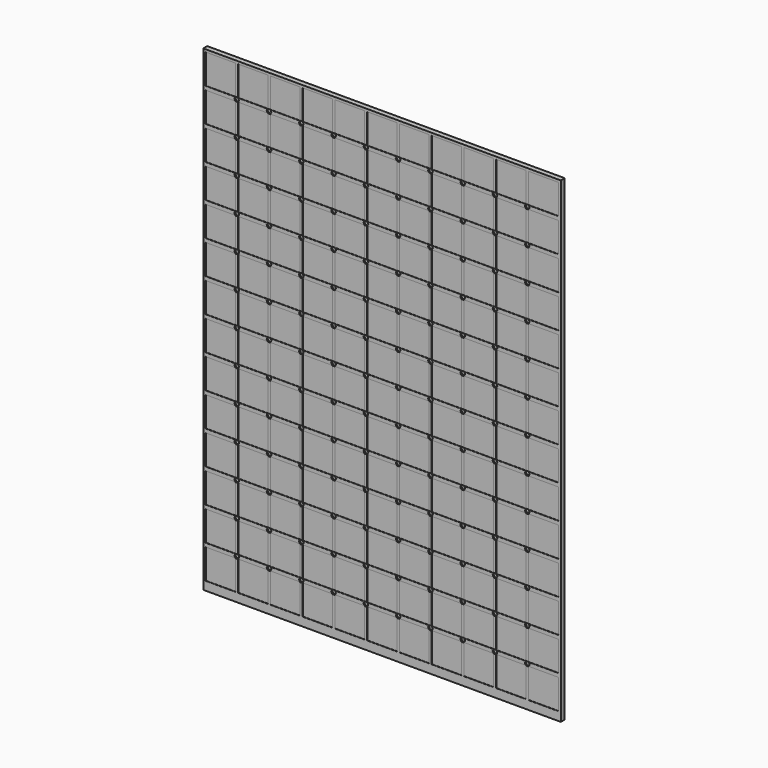
from build123d import *

# Parameters (mm, degrees)
F0_W     = 1828.8
F0_H     = 2438.4
F1_DEPTH = 25.4
F2_W     = 152.4
F2_H     = 152.4
F3_DEPTH = 1.5875
F5_DEPTH = 6.35


# Not quite as in the source:
# - a length typed as a fraction of an inch, garbled in the dataset ("3 / 203.2 mm" for 3/8 in), is restored


with BuildPart() as f1:
    # F0 (on Front) → F1 (new body)
    with BuildSketch(Plane.XZ):
        with Locations((816.0034323931, 1150.0703020215)):
            Rectangle(F0_W, F0_H)
    extrude(amount=F1_DEPTH)

    # F2 (on face) → F3 (cut)
    with BuildSketch(Plane.XZ.offset(25.4)):
        with Locations((-9.4965676069, 2280.3703020215)):
            Rectangle(F2_W, F2_H)
        with Locations((-9.4965676069, 2108.9203020215)):
            Rectangle(F2_W, F2_H)
        with Locations((-9.4965676069, 1937.4703020215)):
            Rectangle(F2_W, F2_H)
        with Locations((-9.4965676069, 1766.0203020215)):
            Rectangle(F2_W, F2_H)
        with Locations((-9.4965676069, 1594.5703020215)):
            Rectangle(F2_W, F2_H)
        with Locations((-9.4965676069, 1423.1203020215)):
            Rectangle(F2_W, F2_H)
        with Locations((-9.4965676069, 1251.6703020215)):
            Rectangle(F2_W, F2_H)
        with Locations((-9.4965676069, 1080.2203020215)):
            Rectangle(F2_W, F2_H)
        with Locations((155.6034323931, 2280.3703020215)):
            Rectangle(F2_W, F2_H)
        with Locations((155.6034323931, 2108.9203020215)):
            Rectangle(F2_W, F2_H)
        with Locations((155.6034323931, 1937.4703020215)):
            Rectangle(F2_W, F2_H)
        with Locations((155.6034323931, 1766.0203020215)):
            Rectangle(F2_W, F2_H)
        with Locations((155.6034323931, 1594.5703020215)):
            Rectangle(F2_W, F2_H)
        with Locations((155.6034323931, 1423.1203020215)):
            Rectangle(F2_W, F2_H)
        with Locations((155.6034323931, 1251.6703020215)):
            Rectangle(F2_W, F2_H)
        with Locations((155.6034323931, 1080.2203020215)):
            Rectangle(F2_W, F2_H)
        with Locations((320.7034323931, 2280.3703020215)):
            Rectangle(F2_W, F2_H)
        with Locations((320.7034323931, 2108.9203020215)):
            Rectangle(F2_W, F2_H)
        with Locations((320.7034323931, 1937.4703020215)):
            Rectangle(F2_W, F2_H)
        with Locations((320.7034323931, 1766.0203020215)):
            Rectangle(F2_W, F2_H)
        with Locations((320.7034323931, 1594.5703020215)):
            Rectangle(F2_W, F2_H)
        with Locations((320.7034323931, 1423.1203020215)):
            Rectangle(F2_W, F2_H)
        with Locations((320.7034323931, 1251.6703020215)):
            Rectangle(F2_W, F2_H)
        with Locations((320.7034323931, 1080.2203020215)):
            Rectangle(F2_W, F2_H)
        with Locations((485.8034323931, 2280.3703020215)):
            Rectangle(F2_W, F2_H)
        with Locations((485.8034323931, 2108.9203020215)):
            Rectangle(F2_W, F2_H)
        with Locations((485.8034323931, 1937.4703020215)):
            Rectangle(F2_W, F2_H)
        with Locations((485.8034323931, 1766.0203020215)):
            Rectangle(F2_W, F2_H)
        with Locations((485.8034323931, 1594.5703020215)):
            Rectangle(F2_W, F2_H)
        with Locations((485.8034323931, 1423.1203020215)):
            Rectangle(F2_W, F2_H)
        with Locations((485.8034323931, 1251.6703020215)):
            Rectangle(F2_W, F2_H)
        with Locations((485.8034323931, 1080.2203020215)):
            Rectangle(F2_W, F2_H)
        with Locations((650.9034323931, 2280.3703020215)):
            Rectangle(F2_W, F2_H)
        with Locations((650.9034323931, 2108.9203020215)):
            Rectangle(F2_W, F2_H)
        with Locations((650.9034323931, 1937.4703020215)):
            Rectangle(F2_W, F2_H)
        with Locations((650.9034323931, 1766.0203020215)):
            Rectangle(F2_W, F2_H)
        with Locations((650.9034323931, 1594.5703020215)):
            Rectangle(F2_W, F2_H)
        with Locations((650.9034323931, 1423.1203020215)):
            Rectangle(F2_W, F2_H)
        with Locations((650.9034323931, 1251.6703020215)):
            Rectangle(F2_W, F2_H)
        with Locations((650.9034323931, 1080.2203020215)):
            Rectangle(F2_W, F2_H)
        with Locations((816.0034323931, 2280.3703020215)):
            Rectangle(F2_W, F2_H)
        with Locations((816.0034323931, 2108.9203020215)):
            Rectangle(F2_W, F2_H)
        with Locations((816.0034323931, 1937.4703020215)):
            Rectangle(F2_W, F2_H)
        with Locations((816.0034323931, 1766.0203020215)):
            Rectangle(F2_W, F2_H)
        with Locations((816.0034323931, 1594.5703020215)):
            Rectangle(F2_W, F2_H)
        with Locations((816.0034323931, 1423.1203020215)):
            Rectangle(F2_W, F2_H)
        with Locations((816.0034323931, 1251.6703020215)):
            Rectangle(F2_W, F2_H)
        with Locations((816.0034323931, 1080.2203020215)):
            Rectangle(F2_W, F2_H)
        with Locations((981.1034323931, 2280.3703020215)):
            Rectangle(F2_W, F2_H)
        with Locations((981.1034323931, 2108.9203020215)):
            Rectangle(F2_W, F2_H)
        with Locations((981.1034323931, 1937.4703020215)):
            Rectangle(F2_W, F2_H)
        with Locations((981.1034323931, 1766.0203020215)):
            Rectangle(F2_W, F2_H)
        with Locations((981.1034323931, 1594.5703020215)):
            Rectangle(F2_W, F2_H)
        with Locations((981.1034323931, 1423.1203020215)):
            Rectangle(F2_W, F2_H)
        with Locations((981.1034323931, 1251.6703020215)):
            Rectangle(F2_W, F2_H)
        with Locations((981.1034323931, 1080.2203020215)):
            Rectangle(F2_W, F2_H)
        with Locations((-9.4965676069, 908.7703020215)):
            Rectangle(F2_W, F2_H)
        with Locations((155.6034323931, 908.7703020215)):
            Rectangle(F2_W, F2_H)
        with Locations((320.7034323931, 908.7703020215)):
            Rectangle(F2_W, F2_H)
        with Locations((485.8034323931, 908.7703020215)):
            Rectangle(F2_W, F2_H)
        with Locations((650.9034323931, 908.7703020215)):
            Rectangle(F2_W, F2_H)
        with Locations((816.0034323931, 908.7703020215)):
            Rectangle(F2_W, F2_H)
        with Locations((981.1034323931, 908.7703020215)):
            Rectangle(F2_W, F2_H)
        with Locations((1146.2034323931, 2280.3703020215)):
            Rectangle(F2_W, F2_H)
        with Locations((1146.2034323931, 2108.9203020215)):
            Rectangle(F2_W, F2_H)
        with Locations((1146.2034323931, 1937.4703020215)):
            Rectangle(F2_W, F2_H)
        with Locations((1146.2034323931, 1766.0203020215)):
            Rectangle(F2_W, F2_H)
        with Locations((1146.2034323931, 1594.5703020215)):
            Rectangle(F2_W, F2_H)
        with Locations((1146.2034323931, 1423.1203020215)):
            Rectangle(F2_W, F2_H)
        with Locations((1146.2034323931, 1251.6703020215)):
            Rectangle(F2_W, F2_H)
        with Locations((1146.2034323931, 1080.2203020215)):
            Rectangle(F2_W, F2_H)
        with Locations((1146.2034323931, 908.7703020215)):
            Rectangle(F2_W, F2_H)
        with Locations((1311.3034323931, 2280.3703020215)):
            Rectangle(F2_W, F2_H)
        with Locations((1311.3034323931, 2108.9203020215)):
            Rectangle(F2_W, F2_H)
        with Locations((1311.3034323931, 1937.4703020215)):
            Rectangle(F2_W, F2_H)
        with Locations((1311.3034323931, 1766.0203020215)):
            Rectangle(F2_W, F2_H)
        with Locations((1311.3034323931, 1594.5703020215)):
            Rectangle(F2_W, F2_H)
        with Locations((1311.3034323931, 1423.1203020215)):
            Rectangle(F2_W, F2_H)
        with Locations((1311.3034323931, 1251.6703020215)):
            Rectangle(F2_W, F2_H)
        with Locations((1311.3034323931, 1080.2203020215)):
            Rectangle(F2_W, F2_H)
        with Locations((1311.3034323931, 908.7703020215)):
            Rectangle(F2_W, F2_H)
        with Locations((1476.4034323931, 2280.3703020215)):
            Rectangle(F2_W, F2_H)
        with Locations((1476.4034323931, 2108.9203020215)):
            Rectangle(F2_W, F2_H)
        with Locations((1476.4034323931, 1937.4703020215)):
            Rectangle(F2_W, F2_H)
        with Locations((1476.4034323931, 1766.0203020215)):
            Rectangle(F2_W, F2_H)
        with Locations((1476.4034323931, 1594.5703020215)):
            Rectangle(F2_W, F2_H)
        with Locations((1476.4034323931, 1423.1203020215)):
            Rectangle(F2_W, F2_H)
        with Locations((1476.4034323931, 1251.6703020215)):
            Rectangle(F2_W, F2_H)
        with Locations((1476.4034323931, 1080.2203020215)):
            Rectangle(F2_W, F2_H)
        with Locations((1476.4034323931, 908.7703020215)):
            Rectangle(F2_W, F2_H)
        with Locations((1641.5034323931, 2280.3703020215)):
            Rectangle(F2_W, F2_H)
        with Locations((1641.5034323931, 2108.9203020215)):
            Rectangle(F2_W, F2_H)
        with Locations((1641.5034323931, 1937.4703020215)):
            Rectangle(F2_W, F2_H)
        with Locations((1641.5034323931, 1766.0203020215)):
            Rectangle(F2_W, F2_H)
        with Locations((1641.5034323931, 1594.5703020215)):
            Rectangle(F2_W, F2_H)
        with Locations((1641.5034323931, 1423.1203020215)):
            Rectangle(F2_W, F2_H)
        with Locations((1641.5034323931, 1251.6703020215)):
            Rectangle(F2_W, F2_H)
        with Locations((1641.5034323931, 1080.2203020215)):
            Rectangle(F2_W, F2_H)
        with Locations((1641.5034323931, 908.7703020215)):
            Rectangle(F2_W, F2_H)
        with Locations((-9.4965676069, 737.3203020215)):
            Rectangle(F2_W, F2_H)
        with Locations((-9.4965676069, 565.8703020215)):
            Rectangle(F2_W, F2_H)
        with Locations((-9.4965676069, 394.4203020215)):
            Rectangle(F2_W, F2_H)
        with Locations((-9.4965676069, 222.9703020215)):
            Rectangle(F2_W, F2_H)
        with Locations((-9.4965676069, 51.5203020215)):
            Rectangle(F2_W, F2_H)
        with Locations((155.6034323931, 737.3203020215)):
            Rectangle(F2_W, F2_H)
        with Locations((155.6034323931, 565.8703020215)):
            Rectangle(F2_W, F2_H)
        with Locations((155.6034323931, 394.4203020215)):
            Rectangle(F2_W, F2_H)
        with Locations((155.6034323931, 222.9703020215)):
            Rectangle(F2_W, F2_H)
        with Locations((155.6034323931, 51.5203020215)):
            Rectangle(F2_W, F2_H)
        with Locations((320.7034323931, 737.3203020215)):
            Rectangle(F2_W, F2_H)
        with Locations((320.7034323931, 565.8703020215)):
            Rectangle(F2_W, F2_H)
        with Locations((320.7034323931, 394.4203020215)):
            Rectangle(F2_W, F2_H)
        with Locations((320.7034323931, 222.9703020215)):
            Rectangle(F2_W, F2_H)
        with Locations((320.7034323931, 51.5203020215)):
            Rectangle(F2_W, F2_H)
        with Locations((485.8034323931, 737.3203020215)):
            Rectangle(F2_W, F2_H)
        with Locations((485.8034323931, 565.8703020215)):
            Rectangle(F2_W, F2_H)
        with Locations((485.8034323931, 394.4203020215)):
            Rectangle(F2_W, F2_H)
        with Locations((485.8034323931, 222.9703020215)):
            Rectangle(F2_W, F2_H)
        with Locations((485.8034323931, 51.5203020215)):
            Rectangle(F2_W, F2_H)
        with Locations((650.9034323931, 737.3203020215)):
            Rectangle(F2_W, F2_H)
        with Locations((650.9034323931, 565.8703020215)):
            Rectangle(F2_W, F2_H)
        with Locations((650.9034323931, 394.4203020215)):
            Rectangle(F2_W, F2_H)
        with Locations((650.9034323931, 222.9703020215)):
            Rectangle(F2_W, F2_H)
        with Locations((650.9034323931, 51.5203020215)):
            Rectangle(F2_W, F2_H)
        with Locations((816.0034323931, 737.3203020215)):
            Rectangle(F2_W, F2_H)
        with Locations((816.0034323931, 565.8703020215)):
            Rectangle(F2_W, F2_H)
        with Locations((816.0034323931, 394.4203020215)):
            Rectangle(F2_W, F2_H)
        with Locations((816.0034323931, 222.9703020215)):
            Rectangle(F2_W, F2_H)
        with Locations((816.0034323931, 51.5203020215)):
            Rectangle(F2_W, F2_H)
        with Locations((981.1034323931, 737.3203020215)):
            Rectangle(F2_W, F2_H)
        with Locations((981.1034323931, 565.8703020215)):
            Rectangle(F2_W, F2_H)
        with Locations((981.1034323931, 394.4203020215)):
            Rectangle(F2_W, F2_H)
        with Locations((981.1034323931, 222.9703020215)):
            Rectangle(F2_W, F2_H)
        with Locations((981.1034323931, 51.5203020215)):
            Rectangle(F2_W, F2_H)
        with Locations((1146.2034323931, 737.3203020215)):
            Rectangle(F2_W, F2_H)
        with Locations((1146.2034323931, 565.8703020215)):
            Rectangle(F2_W, F2_H)
        with Locations((1146.2034323931, 394.4203020215)):
            Rectangle(F2_W, F2_H)
        with Locations((1146.2034323931, 222.9703020215)):
            Rectangle(F2_W, F2_H)
        with Locations((1146.2034323931, 51.5203020215)):
            Rectangle(F2_W, F2_H)
        with Locations((1311.3034323931, 737.3203020215)):
            Rectangle(F2_W, F2_H)
        with Locations((1311.3034323931, 565.8703020215)):
            Rectangle(F2_W, F2_H)
        with Locations((1311.3034323931, 394.4203020215)):
            Rectangle(F2_W, F2_H)
        with Locations((1311.3034323931, 222.9703020215)):
            Rectangle(F2_W, F2_H)
        with Locations((1311.3034323931, 51.5203020215)):
            Rectangle(F2_W, F2_H)
        with Locations((1476.4034323931, 737.3203020215)):
            Rectangle(F2_W, F2_H)
        with Locations((1476.4034323931, 565.8703020215)):
            Rectangle(F2_W, F2_H)
        with Locations((1476.4034323931, 394.4203020215)):
            Rectangle(F2_W, F2_H)
        with Locations((1476.4034323931, 222.9703020215)):
            Rectangle(F2_W, F2_H)
        with Locations((1476.4034323931, 51.5203020215)):
            Rectangle(F2_W, F2_H)
        with Locations((1641.5034323931, 737.3203020215)):
            Rectangle(F2_W, F2_H)
        with Locations((1641.5034323931, 565.8703020215)):
            Rectangle(F2_W, F2_H)
        with Locations((1641.5034323931, 394.4203020215)):
            Rectangle(F2_W, F2_H)
        with Locations((1641.5034323931, 222.9703020215)):
            Rectangle(F2_W, F2_H)
        with Locations((1641.5034323931, 51.5203020215)):
            Rectangle(F2_W, F2_H)
    extrude(amount=-F3_DEPTH, mode=Mode.SUBTRACT)

    # F4 (on face) → F5 (cut)
    with BuildSketch(Plane.XZ.offset(25.4)):
        Polygon((66.8225524701, 2183.8503020215), (79.2843123161, 2183.8503020215), (85.5151922391, 2194.642502624), (79.2843123161, 2205.4347032265), (66.8225524701, 2205.4347032265), (60.5916725471, 2194.642502624), align=None)
        Polygon((79.2843123161, 2033.9847032265), (66.8225524701, 2033.9847032265), (60.5916725471, 2023.192502624), (66.8225524701, 2012.4003020215), (79.2843123161, 2012.4003020215), (85.5151922391, 2023.192502624), align=None)
        Polygon((79.2843123161, 1862.5347032265), (66.8225524701, 1862.5347032265), (60.5916725471, 1851.742502624), (66.8225524701, 1840.9503020215), (79.2843123161, 1840.9503020215), (85.5151922391, 1851.742502624), align=None)
        Polygon((79.2843123161, 1691.0847032265), (66.8225524701, 1691.0847032265), (60.5916725471, 1680.292502624), (66.8225524701, 1669.5003020215), (79.2843123161, 1669.5003020215), (85.5151922391, 1680.292502624), align=None)
        Polygon((79.2843123161, 1519.6347032265), (66.8225524701, 1519.6347032265), (60.5916725471, 1508.842502624), (66.8225524701, 1498.0503020215), (79.2843123161, 1498.0503020215), (85.5151922391, 1508.842502624), align=None)
        Polygon((79.2843123161, 1348.1847032265), (66.8225524701, 1348.1847032265), (60.5916725471, 1337.392502624), (66.8225524701, 1326.6003020215), (79.2843123161, 1326.6003020215), (85.5151922391, 1337.392502624), align=None)
        Polygon((79.2843123161, 1176.7347032265), (66.8225524701, 1176.7347032265), (60.5916725471, 1165.942502624), (66.8225524701, 1155.1503020215), (79.2843123161, 1155.1503020215), (85.5151922391, 1165.942502624), align=None)
        Polygon((79.2843123161, 1005.2847032265), (66.8225524701, 1005.2847032265), (60.5916725471, 994.492502624), (66.8225524701, 983.7003020215), (79.2843123161, 983.7003020215), (85.5151922391, 994.492502624), align=None)
        Polygon((244.3843123161, 2205.4347032265), (231.9225524701, 2205.4347032265), (225.6916725471, 2194.642502624), (231.9225524701, 2183.8503020215), (244.3843123161, 2183.8503020215), (250.6151922391, 2194.642502624), align=None)
        Polygon((244.3843123161, 2033.9847032265), (231.9225524701, 2033.9847032265), (225.6916725471, 2023.192502624), (231.9225524701, 2012.4003020215), (244.3843123161, 2012.4003020215), (250.6151922391, 2023.192502624), align=None)
        Polygon((244.3843123161, 1862.5347032265), (231.9225524701, 1862.5347032265), (225.6916725471, 1851.742502624), (231.9225524701, 1840.9503020215), (244.3843123161, 1840.9503020215), (250.6151922391, 1851.742502624), align=None)
        Polygon((244.3843123161, 1691.0847032265), (231.9225524701, 1691.0847032265), (225.6916725471, 1680.292502624), (231.9225524701, 1669.5003020215), (244.3843123161, 1669.5003020215), (250.6151922391, 1680.292502624), align=None)
        Polygon((244.3843123161, 1519.6347032265), (231.9225524701, 1519.6347032265), (225.6916725471, 1508.842502624), (231.9225524701, 1498.0503020215), (244.3843123161, 1498.0503020215), (250.6151922391, 1508.842502624), align=None)
        Polygon((244.3843123161, 1348.1847032265), (231.9225524701, 1348.1847032265), (225.6916725471, 1337.392502624), (231.9225524701, 1326.6003020215), (244.3843123161, 1326.6003020215), (250.6151922391, 1337.392502624), align=None)
        Polygon((244.3843123161, 1176.7347032265), (231.9225524701, 1176.7347032265), (225.6916725471, 1165.942502624), (231.9225524701, 1155.1503020215), (244.3843123161, 1155.1503020215), (250.6151922391, 1165.942502624), align=None)
        Polygon((244.3843123161, 1005.2847032265), (231.9225524701, 1005.2847032265), (225.6916725471, 994.492502624), (231.9225524701, 983.7003020215), (244.3843123161, 983.7003020215), (250.6151922391, 994.492502624), align=None)
        Polygon((409.4843123161, 2205.4347032265), (397.0225524701, 2205.4347032265), (390.7916725471, 2194.642502624), (397.0225524701, 2183.8503020215), (409.4843123161, 2183.8503020215), (415.7151922391, 2194.642502624), align=None)
        Polygon((409.4843123161, 2033.9847032265), (397.0225524701, 2033.9847032265), (390.7916725471, 2023.192502624), (397.0225524701, 2012.4003020215), (409.4843123161, 2012.4003020215), (415.7151922391, 2023.192502624), align=None)
        Polygon((409.4843123161, 1862.5347032265), (397.0225524701, 1862.5347032265), (390.7916725471, 1851.742502624), (397.0225524701, 1840.9503020215), (409.4843123161, 1840.9503020215), (415.7151922391, 1851.742502624), align=None)
        Polygon((409.4843123161, 1691.0847032265), (397.0225524701, 1691.0847032265), (390.7916725471, 1680.292502624), (397.0225524701, 1669.5003020215), (409.4843123161, 1669.5003020215), (415.7151922391, 1680.292502624), align=None)
        Polygon((409.4843123161, 1519.6347032265), (397.0225524701, 1519.6347032265), (390.7916725471, 1508.842502624), (397.0225524701, 1498.0503020215), (409.4843123161, 1498.0503020215), (415.7151922391, 1508.842502624), align=None)
        Polygon((409.4843123161, 1348.1847032265), (397.0225524701, 1348.1847032265), (390.7916725471, 1337.392502624), (397.0225524701, 1326.6003020215), (409.4843123161, 1326.6003020215), (415.7151922391, 1337.392502624), align=None)
        Polygon((409.4843123161, 1176.7347032265), (397.0225524701, 1176.7347032265), (390.7916725471, 1165.942502624), (397.0225524701, 1155.1503020215), (409.4843123161, 1155.1503020215), (415.7151922391, 1165.942502624), align=None)
        Polygon((409.4843123161, 1005.2847032265), (397.0225524701, 1005.2847032265), (390.7916725471, 994.492502624), (397.0225524701, 983.7003020215), (409.4843123161, 983.7003020215), (415.7151922391, 994.492502624), align=None)
        Polygon((574.5843123161, 2205.4347032265), (562.1225524701, 2205.4347032265), (555.8916725471, 2194.642502624), (562.1225524701, 2183.8503020215), (574.5843123161, 2183.8503020215), (580.8151922391, 2194.642502624), align=None)
        Polygon((574.5843123161, 2033.9847032265), (562.1225524701, 2033.9847032265), (555.8916725471, 2023.192502624), (562.1225524701, 2012.4003020215), (574.5843123161, 2012.4003020215), (580.8151922391, 2023.192502624), align=None)
        Polygon((574.5843123161, 1862.5347032265), (562.1225524701, 1862.5347032265), (555.8916725471, 1851.742502624), (562.1225524701, 1840.9503020215), (574.5843123161, 1840.9503020215), (580.8151922391, 1851.742502624), align=None)
        Polygon((574.5843123161, 1691.0847032265), (562.1225524701, 1691.0847032265), (555.8916725471, 1680.292502624), (562.1225524701, 1669.5003020215), (574.5843123161, 1669.5003020215), (580.8151922391, 1680.292502624), align=None)
        Polygon((574.5843123161, 1519.6347032265), (562.1225524701, 1519.6347032265), (555.8916725471, 1508.842502624), (562.1225524701, 1498.0503020215), (574.5843123161, 1498.0503020215), (580.8151922391, 1508.842502624), align=None)
        Polygon((574.5843123161, 1348.1847032265), (562.1225524701, 1348.1847032265), (555.8916725471, 1337.392502624), (562.1225524701, 1326.6003020215), (574.5843123161, 1326.6003020215), (580.8151922391, 1337.392502624), align=None)
        Polygon((574.5843123161, 1176.7347032265), (562.1225524701, 1176.7347032265), (555.8916725471, 1165.942502624), (562.1225524701, 1155.1503020215), (574.5843123161, 1155.1503020215), (580.8151922391, 1165.942502624), align=None)
        Polygon((574.5843123161, 1005.2847032265), (562.1225524701, 1005.2847032265), (555.8916725471, 994.492502624), (562.1225524701, 983.7003020215), (574.5843123161, 983.7003020215), (580.8151922391, 994.492502624), align=None)
        Polygon((739.6843123161, 2205.4347032265), (727.2225524701, 2205.4347032265), (720.9916725471, 2194.642502624), (727.2225524701, 2183.8503020215), (739.6843123161, 2183.8503020215), (745.9151922391, 2194.642502624), align=None)
        Polygon((739.6843123161, 2033.9847032265), (727.2225524701, 2033.9847032265), (720.9916725471, 2023.192502624), (727.2225524701, 2012.4003020215), (739.6843123161, 2012.4003020215), (745.9151922391, 2023.192502624), align=None)
        Polygon((739.6843123161, 1862.5347032265), (727.2225524701, 1862.5347032265), (720.9916725471, 1851.742502624), (727.2225524701, 1840.9503020215), (739.6843123161, 1840.9503020215), (745.9151922391, 1851.742502624), align=None)
        Polygon((739.6843123161, 1691.0847032265), (727.2225524701, 1691.0847032265), (720.9916725471, 1680.292502624), (727.2225524701, 1669.5003020215), (739.6843123161, 1669.5003020215), (745.9151922391, 1680.292502624), align=None)
        Polygon((739.6843123161, 1519.6347032265), (727.2225524701, 1519.6347032265), (720.9916725471, 1508.842502624), (727.2225524701, 1498.0503020215), (739.6843123161, 1498.0503020215), (745.9151922391, 1508.842502624), align=None)
        Polygon((739.6843123161, 1348.1847032265), (727.2225524701, 1348.1847032265), (720.9916725471, 1337.392502624), (727.2225524701, 1326.6003020215), (739.6843123161, 1326.6003020215), (745.9151922391, 1337.392502624), align=None)
        Polygon((739.6843123161, 1176.7347032265), (727.2225524701, 1176.7347032265), (720.9916725471, 1165.942502624), (727.2225524701, 1155.1503020215), (739.6843123161, 1155.1503020215), (745.9151922391, 1165.942502624), align=None)
        Polygon((739.6843123161, 1005.2847032265), (727.2225524701, 1005.2847032265), (720.9916725471, 994.492502624), (727.2225524701, 983.7003020215), (739.6843123161, 983.7003020215), (745.9151922391, 994.492502624), align=None)
        Polygon((904.7843123161, 2205.4347032265), (892.3225524701, 2205.4347032265), (886.0916725471, 2194.642502624), (892.3225524701, 2183.8503020215), (904.7843123161, 2183.8503020215), (911.0151922391, 2194.642502624), align=None)
        Polygon((904.7843123161, 2033.9847032265), (892.3225524701, 2033.9847032265), (886.0916725471, 2023.192502624), (892.3225524701, 2012.4003020215), (904.7843123161, 2012.4003020215), (911.0151922391, 2023.192502624), align=None)
        Polygon((904.7843123161, 1862.5347032265), (892.3225524701, 1862.5347032265), (886.0916725471, 1851.742502624), (892.3225524701, 1840.9503020215), (904.7843123161, 1840.9503020215), (911.0151922391, 1851.742502624), align=None)
        Polygon((904.7843123161, 1691.0847032265), (892.3225524701, 1691.0847032265), (886.0916725471, 1680.292502624), (892.3225524701, 1669.5003020215), (904.7843123161, 1669.5003020215), (911.0151922391, 1680.292502624), align=None)
        Polygon((904.7843123161, 1519.6347032265), (892.3225524701, 1519.6347032265), (886.0916725471, 1508.842502624), (892.3225524701, 1498.0503020215), (904.7843123161, 1498.0503020215), (911.0151922391, 1508.842502624), align=None)
        Polygon((904.7843123161, 1348.1847032265), (892.3225524701, 1348.1847032265), (886.0916725471, 1337.392502624), (892.3225524701, 1326.6003020215), (904.7843123161, 1326.6003020215), (911.0151922391, 1337.392502624), align=None)
        Polygon((904.7843123161, 1176.7347032265), (892.3225524701, 1176.7347032265), (886.0916725471, 1165.942502624), (892.3225524701, 1155.1503020215), (904.7843123161, 1155.1503020215), (911.0151922391, 1165.942502624), align=None)
        Polygon((904.7843123161, 1005.2847032265), (892.3225524701, 1005.2847032265), (886.0916725471, 994.492502624), (892.3225524701, 983.7003020215), (904.7843123161, 983.7003020215), (911.0151922391, 994.492502624), align=None)
        Polygon((1069.8843123161, 2205.4347032265), (1057.4225524701, 2205.4347032265), (1051.1916725471, 2194.642502624), (1057.4225524701, 2183.8503020215), (1069.8843123161, 2183.8503020215), (1076.1151922391, 2194.642502624), align=None)
        Polygon((1069.8843123161, 2033.9847032265), (1057.4225524701, 2033.9847032265), (1051.1916725471, 2023.192502624), (1057.4225524701, 2012.4003020215), (1069.8843123161, 2012.4003020215), (1076.1151922391, 2023.192502624), align=None)
        Polygon((1069.8843123161, 1862.5347032265), (1057.4225524701, 1862.5347032265), (1051.1916725471, 1851.742502624), (1057.4225524701, 1840.9503020215), (1069.8843123161, 1840.9503020215), (1076.1151922391, 1851.742502624), align=None)
        Polygon((1069.8843123161, 1691.0847032265), (1057.4225524701, 1691.0847032265), (1051.1916725471, 1680.292502624), (1057.4225524701, 1669.5003020215), (1069.8843123161, 1669.5003020215), (1076.1151922391, 1680.292502624), align=None)
        Polygon((1069.8843123161, 1519.6347032265), (1057.4225524701, 1519.6347032265), (1051.1916725471, 1508.842502624), (1057.4225524701, 1498.0503020215), (1069.8843123161, 1498.0503020215), (1076.1151922391, 1508.842502624), align=None)
        Polygon((1069.8843123161, 1348.1847032265), (1057.4225524701, 1348.1847032265), (1051.1916725471, 1337.392502624), (1057.4225524701, 1326.6003020215), (1069.8843123161, 1326.6003020215), (1076.1151922391, 1337.392502624), align=None)
        Polygon((1069.8843123161, 1176.7347032265), (1057.4225524701, 1176.7347032265), (1051.1916725471, 1165.942502624), (1057.4225524701, 1155.1503020215), (1069.8843123161, 1155.1503020215), (1076.1151922391, 1165.942502624), align=None)
        Polygon((1069.8843123161, 1005.2847032265), (1057.4225524701, 1005.2847032265), (1051.1916725471, 994.492502624), (1057.4225524701, 983.7003020215), (1069.8843123161, 983.7003020215), (1076.1151922391, 994.492502624), align=None)
        Polygon((1234.9843123161, 2205.4347032265), (1222.5225524701, 2205.4347032265), (1216.2916725471, 2194.642502624), (1222.5225524701, 2183.8503020215), (1234.9843123161, 2183.8503020215), (1241.2151922391, 2194.642502624), align=None)
        Polygon((1234.9843123161, 2033.9847032265), (1222.5225524701, 2033.9847032265), (1216.2916725471, 2023.192502624), (1222.5225524701, 2012.4003020215), (1234.9843123161, 2012.4003020215), (1241.2151922391, 2023.192502624), align=None)
        Polygon((1234.9843123161, 1862.5347032265), (1222.5225524701, 1862.5347032265), (1216.2916725471, 1851.742502624), (1222.5225524701, 1840.9503020215), (1234.9843123161, 1840.9503020215), (1241.2151922391, 1851.742502624), align=None)
        Polygon((1234.9843123161, 1691.0847032265), (1222.5225524701, 1691.0847032265), (1216.2916725471, 1680.292502624), (1222.5225524701, 1669.5003020215), (1234.9843123161, 1669.5003020215), (1241.2151922391, 1680.292502624), align=None)
        Polygon((1234.9843123161, 1519.6347032265), (1222.5225524701, 1519.6347032265), (1216.2916725471, 1508.842502624), (1222.5225524701, 1498.0503020215), (1234.9843123161, 1498.0503020215), (1241.2151922391, 1508.842502624), align=None)
        Polygon((1234.9843123161, 1348.1847032265), (1222.5225524701, 1348.1847032265), (1216.2916725471, 1337.392502624), (1222.5225524701, 1326.6003020215), (1234.9843123161, 1326.6003020215), (1241.2151922391, 1337.392502624), align=None)
        Polygon((1234.9843123161, 1176.7347032265), (1222.5225524701, 1176.7347032265), (1216.2916725471, 1165.942502624), (1222.5225524701, 1155.1503020215), (1234.9843123161, 1155.1503020215), (1241.2151922391, 1165.942502624), align=None)
        Polygon((1234.9843123161, 1005.2847032265), (1222.5225524701, 1005.2847032265), (1216.2916725471, 994.492502624), (1222.5225524701, 983.7003020215), (1234.9843123161, 983.7003020215), (1241.2151922391, 994.492502624), align=None)
        Polygon((1400.0843123161, 2205.4347032265), (1387.6225524701, 2205.4347032265), (1381.3916725471, 2194.642502624), (1387.6225524701, 2183.8503020215), (1400.0843123161, 2183.8503020215), (1406.3151922391, 2194.642502624), align=None)
        Polygon((1400.0843123161, 2033.9847032265), (1387.6225524701, 2033.9847032265), (1381.3916725471, 2023.192502624), (1387.6225524701, 2012.4003020215), (1400.0843123161, 2012.4003020215), (1406.3151922391, 2023.192502624), align=None)
        Polygon((1400.0843123161, 1862.5347032265), (1387.6225524701, 1862.5347032265), (1381.3916725471, 1851.742502624), (1387.6225524701, 1840.9503020215), (1400.0843123161, 1840.9503020215), (1406.3151922391, 1851.742502624), align=None)
        Polygon((1400.0843123161, 1691.0847032265), (1387.6225524701, 1691.0847032265), (1381.3916725471, 1680.292502624), (1387.6225524701, 1669.5003020215), (1400.0843123161, 1669.5003020215), (1406.3151922391, 1680.292502624), align=None)
        Polygon((1400.0843123161, 1519.6347032265), (1387.6225524701, 1519.6347032265), (1381.3916725471, 1508.842502624), (1387.6225524701, 1498.0503020215), (1400.0843123161, 1498.0503020215), (1406.3151922391, 1508.842502624), align=None)
        Polygon((1400.0843123161, 1348.1847032265), (1387.6225524701, 1348.1847032265), (1381.3916725471, 1337.392502624), (1387.6225524701, 1326.6003020215), (1400.0843123161, 1326.6003020215), (1406.3151922391, 1337.392502624), align=None)
        Polygon((1400.0843123161, 1176.7347032265), (1387.6225524701, 1176.7347032265), (1381.3916725471, 1165.942502624), (1387.6225524701, 1155.1503020215), (1400.0843123161, 1155.1503020215), (1406.3151922391, 1165.942502624), align=None)
        Polygon((1400.0843123161, 1005.2847032265), (1387.6225524701, 1005.2847032265), (1381.3916725471, 994.492502624), (1387.6225524701, 983.7003020215), (1400.0843123161, 983.7003020215), (1406.3151922391, 994.492502624), align=None)
        Polygon((1565.1843123161, 2205.4347032265), (1552.7225524701, 2205.4347032265), (1546.4916725471, 2194.642502624), (1552.7225524701, 2183.8503020215), (1565.1843123161, 2183.8503020215), (1571.4151922391, 2194.642502624), align=None)
        Polygon((1565.1843123161, 2033.9847032265), (1552.7225524701, 2033.9847032265), (1546.4916725471, 2023.192502624), (1552.7225524701, 2012.4003020215), (1565.1843123161, 2012.4003020215), (1571.4151922391, 2023.192502624), align=None)
        Polygon((1565.1843123161, 1862.5347032265), (1552.7225524701, 1862.5347032265), (1546.4916725471, 1851.742502624), (1552.7225524701, 1840.9503020215), (1565.1843123161, 1840.9503020215), (1571.4151922391, 1851.742502624), align=None)
        Polygon((1565.1843123161, 1691.0847032265), (1552.7225524701, 1691.0847032265), (1546.4916725471, 1680.292502624), (1552.7225524701, 1669.5003020215), (1565.1843123161, 1669.5003020215), (1571.4151922391, 1680.292502624), align=None)
        Polygon((1565.1843123161, 1519.6347032265), (1552.7225524701, 1519.6347032265), (1546.4916725471, 1508.842502624), (1552.7225524701, 1498.0503020215), (1565.1843123161, 1498.0503020215), (1571.4151922391, 1508.842502624), align=None)
        Polygon((1565.1843123161, 1348.1847032265), (1552.7225524701, 1348.1847032265), (1546.4916725471, 1337.392502624), (1552.7225524701, 1326.6003020215), (1565.1843123161, 1326.6003020215), (1571.4151922391, 1337.392502624), align=None)
        Polygon((1565.1843123161, 1176.7347032265), (1552.7225524701, 1176.7347032265), (1546.4916725471, 1165.942502624), (1552.7225524701, 1155.1503020215), (1565.1843123161, 1155.1503020215), (1571.4151922391, 1165.942502624), align=None)
        Polygon((1565.1843123161, 1005.2847032265), (1552.7225524701, 1005.2847032265), (1546.4916725471, 994.492502624), (1552.7225524701, 983.7003020215), (1565.1843123161, 983.7003020215), (1571.4151922391, 994.492502624), align=None)
        Polygon((79.2843123161, 833.8347032265), (66.8225524701, 833.8347032265), (60.5916725471, 823.042502624), (66.8225524701, 812.2503020215), (79.2843123161, 812.2503020215), (85.5151922391, 823.042502624), align=None)
        Polygon((79.2843123161, 662.3847032265), (66.8225524701, 662.3847032265), (60.5916725471, 651.592502624), (66.8225524701, 640.8003020215), (79.2843123161, 640.8003020215), (85.5151922391, 651.592502624), align=None)
        Polygon((79.2843123161, 490.9347032265), (66.8225524701, 490.9347032265), (60.5916725471, 480.142502624), (66.8225524701, 469.3503020215), (79.2843123161, 469.3503020215), (85.5151922391, 480.142502624), align=None)
        Polygon((79.2843123161, 319.4847032265), (66.8225524701, 319.4847032265), (60.5916725471, 308.692502624), (66.8225524701, 297.9003020215), (79.2843123161, 297.9003020215), (85.5151922391, 308.692502624), align=None)
        Polygon((244.3843123161, 833.8347032265), (231.9225524701, 833.8347032265), (225.6916725471, 823.042502624), (231.9225524701, 812.2503020215), (244.3843123161, 812.2503020215), (250.6151922391, 823.042502624), align=None)
        Polygon((244.3843123161, 662.3847032265), (231.9225524701, 662.3847032265), (225.6916725471, 651.592502624), (231.9225524701, 640.8003020215), (244.3843123161, 640.8003020215), (250.6151922391, 651.592502624), align=None)
        Polygon((244.3843123161, 490.9347032265), (231.9225524701, 490.9347032265), (225.6916725471, 480.142502624), (231.9225524701, 469.3503020215), (244.3843123161, 469.3503020215), (250.6151922391, 480.142502624), align=None)
        Polygon((244.3843123161, 319.4847032265), (231.9225524701, 319.4847032265), (225.6916725471, 308.692502624), (231.9225524701, 297.9003020215), (244.3843123161, 297.9003020215), (250.6151922391, 308.692502624), align=None)
        Polygon((409.4843123161, 833.8347032265), (397.0225524701, 833.8347032265), (390.7916725471, 823.042502624), (397.0225524701, 812.2503020215), (409.4843123161, 812.2503020215), (415.7151922391, 823.042502624), align=None)
        Polygon((409.4843123161, 662.3847032265), (397.0225524701, 662.3847032265), (390.7916725471, 651.592502624), (397.0225524701, 640.8003020215), (409.4843123161, 640.8003020215), (415.7151922391, 651.592502624), align=None)
        Polygon((409.4843123161, 490.9347032265), (397.0225524701, 490.9347032265), (390.7916725471, 480.142502624), (397.0225524701, 469.3503020215), (409.4843123161, 469.3503020215), (415.7151922391, 480.142502624), align=None)
        Polygon((409.4843123161, 319.4847032265), (397.0225524701, 319.4847032265), (390.7916725471, 308.692502624), (397.0225524701, 297.9003020215), (409.4843123161, 297.9003020215), (415.7151922391, 308.692502624), align=None)
        Polygon((574.5843123161, 833.8347032265), (562.1225524701, 833.8347032265), (555.8916725471, 823.042502624), (562.1225524701, 812.2503020215), (574.5843123161, 812.2503020215), (580.8151922391, 823.042502624), align=None)
        Polygon((574.5843123161, 662.3847032265), (562.1225524701, 662.3847032265), (555.8916725471, 651.592502624), (562.1225524701, 640.8003020215), (574.5843123161, 640.8003020215), (580.8151922391, 651.592502624), align=None)
        Polygon((574.5843123161, 490.9347032265), (562.1225524701, 490.9347032265), (555.8916725471, 480.142502624), (562.1225524701, 469.3503020215), (574.5843123161, 469.3503020215), (580.8151922391, 480.142502624), align=None)
        Polygon((574.5843123161, 319.4847032265), (562.1225524701, 319.4847032265), (555.8916725471, 308.692502624), (562.1225524701, 297.9003020215), (574.5843123161, 297.9003020215), (580.8151922391, 308.692502624), align=None)
        Polygon((739.6843123161, 833.8347032265), (727.2225524701, 833.8347032265), (720.9916725471, 823.042502624), (727.2225524701, 812.2503020215), (739.6843123161, 812.2503020215), (745.9151922391, 823.042502624), align=None)
        Polygon((739.6843123161, 662.3847032265), (727.2225524701, 662.3847032265), (720.9916725471, 651.592502624), (727.2225524701, 640.8003020215), (739.6843123161, 640.8003020215), (745.9151922391, 651.592502624), align=None)
        Polygon((739.6843123161, 490.9347032265), (727.2225524701, 490.9347032265), (720.9916725471, 480.142502624), (727.2225524701, 469.3503020215), (739.6843123161, 469.3503020215), (745.9151922391, 480.142502624), align=None)
        Polygon((739.6843123161, 319.4847032265), (727.2225524701, 319.4847032265), (720.9916725471, 308.692502624), (727.2225524701, 297.9003020215), (739.6843123161, 297.9003020215), (745.9151922391, 308.692502624), align=None)
        Polygon((904.7843123161, 833.8347032265), (892.3225524701, 833.8347032265), (886.0916725471, 823.042502624), (892.3225524701, 812.2503020215), (904.7843123161, 812.2503020215), (911.0151922391, 823.042502624), align=None)
        Polygon((904.7843123161, 662.3847032265), (892.3225524701, 662.3847032265), (886.0916725471, 651.592502624), (892.3225524701, 640.8003020215), (904.7843123161, 640.8003020215), (911.0151922391, 651.592502624), align=None)
        Polygon((904.7843123161, 490.9347032265), (892.3225524701, 490.9347032265), (886.0916725471, 480.142502624), (892.3225524701, 469.3503020215), (904.7843123161, 469.3503020215), (911.0151922391, 480.142502624), align=None)
        Polygon((904.7843123161, 319.4847032265), (892.3225524701, 319.4847032265), (886.0916725471, 308.692502624), (892.3225524701, 297.9003020215), (904.7843123161, 297.9003020215), (911.0151922391, 308.692502624), align=None)
        Polygon((1069.8843123161, 833.8347032265), (1057.4225524701, 833.8347032265), (1051.1916725471, 823.042502624), (1057.4225524701, 812.2503020215), (1069.8843123161, 812.2503020215), (1076.1151922391, 823.042502624), align=None)
        Polygon((1069.8843123161, 662.3847032265), (1057.4225524701, 662.3847032265), (1051.1916725471, 651.592502624), (1057.4225524701, 640.8003020215), (1069.8843123161, 640.8003020215), (1076.1151922391, 651.592502624), align=None)
        Polygon((1069.8843123161, 490.9347032265), (1057.4225524701, 490.9347032265), (1051.1916725471, 480.142502624), (1057.4225524701, 469.3503020215), (1069.8843123161, 469.3503020215), (1076.1151922391, 480.142502624), align=None)
        Polygon((1069.8843123161, 319.4847032265), (1057.4225524701, 319.4847032265), (1051.1916725471, 308.692502624), (1057.4225524701, 297.9003020215), (1069.8843123161, 297.9003020215), (1076.1151922391, 308.692502624), align=None)
        Polygon((1234.9843123161, 833.8347032265), (1222.5225524701, 833.8347032265), (1216.2916725471, 823.042502624), (1222.5225524701, 812.2503020215), (1234.9843123161, 812.2503020215), (1241.2151922391, 823.042502624), align=None)
        Polygon((1234.9843123161, 662.3847032265), (1222.5225524701, 662.3847032265), (1216.2916725471, 651.592502624), (1222.5225524701, 640.8003020215), (1234.9843123161, 640.8003020215), (1241.2151922391, 651.592502624), align=None)
        Polygon((1234.9843123161, 490.9347032265), (1222.5225524701, 490.9347032265), (1216.2916725471, 480.142502624), (1222.5225524701, 469.3503020215), (1234.9843123161, 469.3503020215), (1241.2151922391, 480.142502624), align=None)
        Polygon((1234.9843123161, 319.4847032265), (1222.5225524701, 319.4847032265), (1216.2916725471, 308.692502624), (1222.5225524701, 297.9003020215), (1234.9843123161, 297.9003020215), (1241.2151922391, 308.692502624), align=None)
        Polygon((1400.0843123161, 833.8347032265), (1387.6225524701, 833.8347032265), (1381.3916725471, 823.042502624), (1387.6225524701, 812.2503020215), (1400.0843123161, 812.2503020215), (1406.3151922391, 823.042502624), align=None)
        Polygon((1400.0843123161, 662.3847032265), (1387.6225524701, 662.3847032265), (1381.3916725471, 651.592502624), (1387.6225524701, 640.8003020215), (1400.0843123161, 640.8003020215), (1406.3151922391, 651.592502624), align=None)
        Polygon((1400.0843123161, 490.9347032265), (1387.6225524701, 490.9347032265), (1381.3916725471, 480.142502624), (1387.6225524701, 469.3503020215), (1400.0843123161, 469.3503020215), (1406.3151922391, 480.142502624), align=None)
        Polygon((1400.0843123161, 319.4847032265), (1387.6225524701, 319.4847032265), (1381.3916725471, 308.692502624), (1387.6225524701, 297.9003020215), (1400.0843123161, 297.9003020215), (1406.3151922391, 308.692502624), align=None)
        Polygon((1565.1843123161, 833.8347032265), (1552.7225524701, 833.8347032265), (1546.4916725471, 823.042502624), (1552.7225524701, 812.2503020215), (1565.1843123161, 812.2503020215), (1571.4151922391, 823.042502624), align=None)
        Polygon((1565.1843123161, 662.3847032265), (1552.7225524701, 662.3847032265), (1546.4916725471, 651.592502624), (1552.7225524701, 640.8003020215), (1565.1843123161, 640.8003020215), (1571.4151922391, 651.592502624), align=None)
        Polygon((1565.1843123161, 490.9347032265), (1552.7225524701, 490.9347032265), (1546.4916725471, 480.142502624), (1552.7225524701, 469.3503020215), (1565.1843123161, 469.3503020215), (1571.4151922391, 480.142502624), align=None)
        Polygon((1565.1843123161, 319.4847032265), (1552.7225524701, 319.4847032265), (1546.4916725471, 308.692502624), (1552.7225524701, 297.9003020215), (1565.1843123161, 297.9003020215), (1571.4151922391, 308.692502624), align=None)
        Polygon((79.2843123161, 148.0347032265), (66.8225524701, 148.0347032265), (60.5916725471, 137.242502624), (66.8225524701, 126.4503020215), (79.2843123161, 126.4503020215), (85.5151922391, 137.242502624), align=None)
        Polygon((244.3843123161, 148.0347032265), (231.9225524701, 148.0347032265), (225.6916725471, 137.242502624), (231.9225524701, 126.4503020215), (244.3843123161, 126.4503020215), (250.6151922391, 137.242502624), align=None)
        Polygon((409.4843123161, 148.0347032265), (397.0225524701, 148.0347032265), (390.7916725471, 137.242502624), (397.0225524701, 126.4503020215), (409.4843123161, 126.4503020215), (415.7151922391, 137.242502624), align=None)
        Polygon((574.5843123161, 148.0347032265), (562.1225524701, 148.0347032265), (555.8916725471, 137.242502624), (562.1225524701, 126.4503020215), (574.5843123161, 126.4503020215), (580.8151922391, 137.242502624), align=None)
        Polygon((739.6843123161, 148.0347032265), (727.2225524701, 148.0347032265), (720.9916725471, 137.242502624), (727.2225524701, 126.4503020215), (739.6843123161, 126.4503020215), (745.9151922391, 137.242502624), align=None)
        Polygon((904.7843123161, 148.0347032265), (892.3225524701, 148.0347032265), (886.0916725471, 137.242502624), (892.3225524701, 126.4503020215), (904.7843123161, 126.4503020215), (911.0151922391, 137.242502624), align=None)
        Polygon((1069.8843123161, 148.0347032265), (1057.4225524701, 148.0347032265), (1051.1916725471, 137.242502624), (1057.4225524701, 126.4503020215), (1069.8843123161, 126.4503020215), (1076.1151922391, 137.242502624), align=None)
        Polygon((1234.9843123161, 148.0347032265), (1222.5225524701, 148.0347032265), (1216.2916725471, 137.242502624), (1222.5225524701, 126.4503020215), (1234.9843123161, 126.4503020215), (1241.2151922391, 137.242502624), align=None)
        Polygon((1400.0843123161, 148.0347032265), (1387.6225524701, 148.0347032265), (1381.3916725471, 137.242502624), (1387.6225524701, 126.4503020215), (1400.0843123161, 126.4503020215), (1406.3151922391, 137.242502624), align=None)
        Polygon((1565.1843123161, 148.0347032265), (1552.7225524701, 148.0347032265), (1546.4916725471, 137.242502624), (1552.7225524701, 126.4503020215), (1565.1843123161, 126.4503020215), (1571.4151922391, 137.242502624), align=None)
    extrude(amount=-F5_DEPTH, mode=Mode.SUBTRACT)


solid = f1.part
